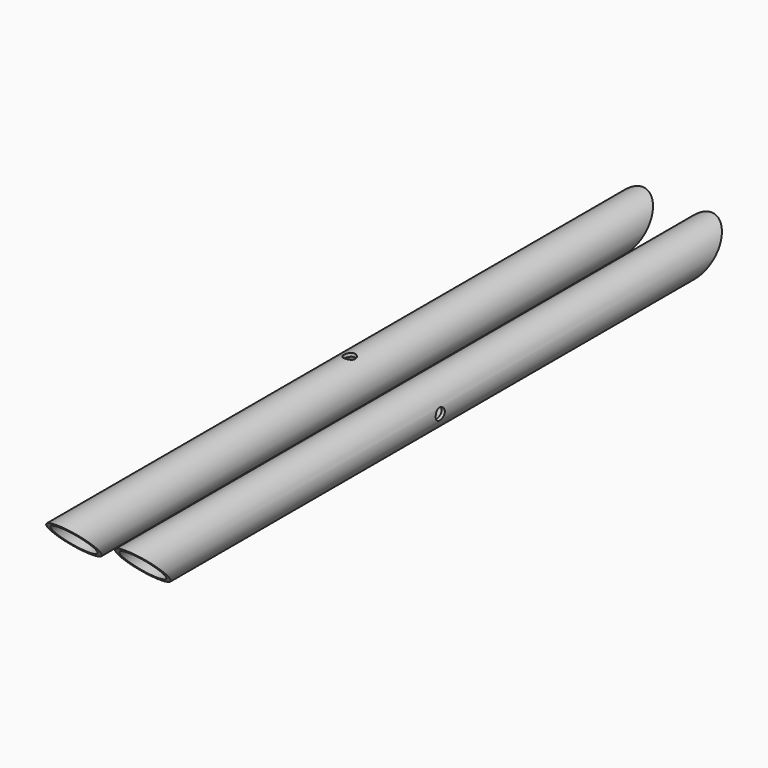
from build123d import *

# Parameters (mm, degrees)
F0_R     = 24.13
F0_R_2   = 20.447
F1_DEPTH = 431.8
F2_R     = 24.13
F2_R_2   = 20.447
F3_DEPTH = 457.2
F5_DEPTH = 152.4
F6_R     = 6.35
F7_DEPTH = 76.2
F8_R     = 6.35
F9_DEPTH = 76.2


with BuildPart() as f1:
    # F0 (on Front) → F1 (new body, symmetric)
    with BuildSketch(Plane.XZ):
        Circle(F0_R)
        Circle(F0_R_2, mode=Mode.SUBTRACT)
    extrude(amount=F1_DEPTH, both=True)


with BuildPart() as f3:
    # F2 (on Front) → F3 (new body, symmetric)
    with BuildSketch(Plane.XZ):
        with Locations((-76.2, 0)):
            Circle(F2_R)
        with Locations((-76.2, 0)):
            Circle(F2_R_2, mode=Mode.SUBTRACT)
    extrude(amount=F3_DEPTH, both=True)


with BuildPart() as f5_tool:
    # F4 (on Right) → F5 (new body, symmetric)
    with BuildSketch(Plane.YZ):
        Polygon((-424.8299507257, 43.8299507257), (-462.2847161403, 104.5060300127), (-486.3353615056, -36.4805202162), (-324.6154958919, -56.3845041081), (-381, 0), align=None)
        Polygon((462.2847161403, 104.5060300127), (424.8299507257, 43.8299507257), (381, 0), (324.6154958919, -56.3845041081), (486.3353615056, -36.4805202162), align=None)
    extrude(amount=F5_DEPTH, both=True)


with BuildPart() as f1_1:
    add(f1.part)

    # F5: cut by f5_tool
    add(f5_tool.part, mode=Mode.SUBTRACT)

    # F6 (on Right) → F7 (cut, symmetric)
    with BuildSketch(Plane.YZ):
        Circle(F6_R)
    extrude(amount=F7_DEPTH, both=True, mode=Mode.SUBTRACT)


with BuildPart() as f3_1:
    add(f3.part)

    # F5: cut by f5_tool
    add(f5_tool.part, mode=Mode.SUBTRACT)

    # F8 (on Top) → F9 (cut, symmetric)
    with BuildSketch(Plane.XY):
        with Locations((-76.2, 0)):
            Circle(F8_R)
    extrude(amount=F9_DEPTH, both=True, mode=Mode.SUBTRACT)


solid = Compound([f1_1.part, f3_1.part])
